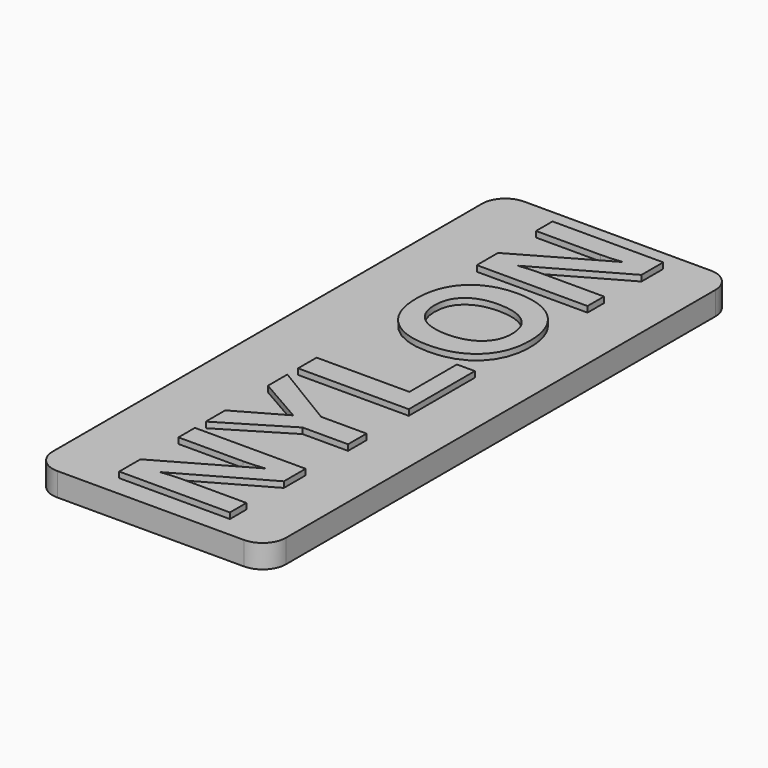
from build123d import *

# Parameters (mm, degrees)
F0_W         = 20
F0_H         = 50
F1_DEPTH     = 2
F2_R         = 2
F3_TEXT_SIZE = 13.7895914829
F4_DEPTH     = 2.5


# Not quite as in the source:
# - Text() gives the source's letters only with a copy of the font that has no kerning and outlines rounded to 1/6400 em; it was checked with that copy


with BuildPart() as f1:
    # F0 (on Top) → F1 (new body)
    with BuildSketch(Plane.XY):
        with Locations((-10, 0)):
            Rectangle(F0_W, F0_H)
    extrude(amount=F1_DEPTH)

    # F2
    f2_edges = [f1.edges().sort_by_distance(p)[0] for p in [
        (0, -25, 1),
        (-20, -25, 1),
        (0, 25, 1),
        (-20, 25, 1),
    ]]
    fillet(f2_edges, radius=F2_R)


with BuildPart() as f4:
    # F3 (on Top) → F4 (new body)
    with BuildSketch(Plane.XY):
        with Locations(Location((-4.6244021505, -24.145790149), (0, 0, 90))):
            Text('NYLON', F3_TEXT_SIZE, font='Arimo', font_style=FontStyle.BOLD, text_align=(TextAlign.LEFT, TextAlign.BOTTOM))
    extrude(amount=F4_DEPTH)


solid = Compound([f1.part, f4.part])
